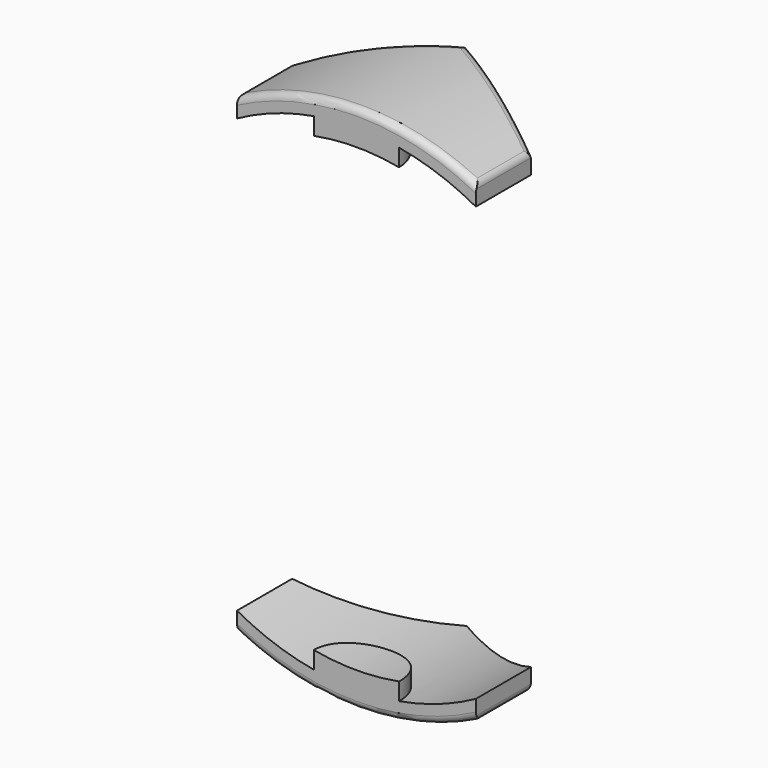
from build123d import *

# Parameters (mm, degrees)
F0_R     = 19.685
F0_R_2   = 18.415
F1_DEPTH = 12.7
F3_DEPTH = 25.4
F4_R     = 3.175
F5_DEPTH = 19.05
F6_R     = 17.145
F7_DEPTH = 12.7
F8_R     = 20.32
F9_DEPTH = 25.4
F10_R    = 0.508


with BuildPart() as f1:
    # F0 (on Front) → F1 (new body, symmetric)
    with BuildSketch(Plane.XZ):
        Circle(F0_R)
        Circle(F0_R_2, mode=Mode.SUBTRACT)
    extrude(amount=F1_DEPTH, both=True)

    # F2 (on Top) → F3 (intersect, symmetric)
    with BuildSketch(Plane.XY):
        Polygon((-8.89, -5.1326438931), (0, -10.2652877862), (8.89, -5.1326438931), (8.89, 5.1326438931), (0, 10.2652877862), (-8.89, 5.1326438931), align=None)
    extrude(amount=F3_DEPTH, both=True, mode=Mode.INTERSECT)

    # F4 (on Top) → F5 (join, symmetric)
    with BuildSketch(Plane.XY):
        Circle(F4_R)
    extrude(amount=F5_DEPTH, both=True)

    # F6 (on Front) → F7 (cut, symmetric)
    with BuildSketch(Plane.XZ):
        Circle(F6_R)
    extrude(amount=F7_DEPTH, both=True, mode=Mode.SUBTRACT)

    # F8 (on Front) → F9 (cut)
    with BuildSketch(Plane.XZ):
        Circle(F8_R)
    extrude(amount=F9_DEPTH, mode=Mode.SUBTRACT)

    # F10
    f10_edges = [f1.edges().sort_by_distance(p)[0] for p in [
        (0, 0, -19.685),
        (0, 0, 19.685),
        (8.89, 2.566322, -17.563232),
        (4.569847, 7.626886, -19.147212),
        (-4.569847, 7.626886, -19.147212),
        (-8.89, 2.566322, -17.563232),
        (-8.89, 2.566322, 17.563232),
        (-4.569847, 7.626886, 19.147212),
        (4.569847, 7.626886, 19.147212),
        (8.89, 2.566322, 17.563232),
    ]]
    fillet(f10_edges, radius=F10_R)


solid = f1.part
